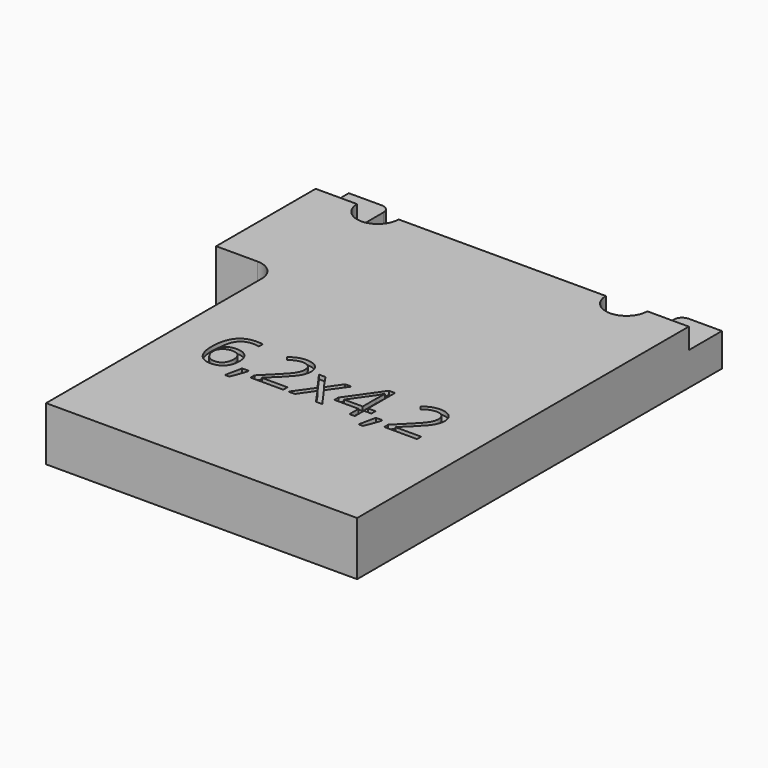
from build123d import *

# Parameters (mm, degrees)
F1_DEPTH     = 13
F2_W         = 107.3082715438
F2_H         = 14.5000026375
F3_DEPTH     = 5
F4_R         = 3
F5_DEPTH     = 10
F6_TEXT_SIZE = 16.861082986
F7_DEPTH     = 1


# Not quite as in the source:
# - Text() gives the source's letters only with a copy of the font that has no kerning and outlines rounded to 1/6400 em; it was checked with that copy


with BuildPart() as f1:
    # F0 (on Top) → F1 (new body)
    with BuildSketch(Plane.XY):
        with BuildLine():
            Line((-42.4800007343, 29.9199996144), (-42.4800007343, -10.0800003856))
            Line((-42.4800007343, -10.0800003856), (-32.5100003928, -10.0800003856))
            ThreePointArc((-32.5100003928, -10.0800003856), (-28.9744664869, -11.5444664797), (-27.5100003928, -15.0800003856))
            Line((-27.5100003928, -15.0800003856), (-27.5100003928, -80.0800003856))
            Line((-27.5100003928, -80.0800003856), (47.5199992657, -80.0800003856))
            Line((47.5199992657, -80.0800003856), (47.5199992657, 29.9199996144))
            Line((47.5199992657, 29.9199996144), (39.5199992657, 29.9199996144))
            ThreePointArc((39.5199992657, 29.9199996144), (38.1057857033, 29.3342131767), (37.5199992657, 27.9199996144))
            Line((37.5199992657, 27.9199996144), (37.5199992657, 19.9199996144))
            ThreePointArc((37.5199992657, 19.9199996144), (32.5199992657, 14.9199996144), (27.5199992657, 19.9199996144))
            Line((27.5199992657, 19.9199996144), (-22.4800007343, 19.9199996144))
            ThreePointArc((-22.4800007343, 19.9199996144), (-27.4800007343, 14.9199996144), (-32.4800007343, 19.9199996144))
            Line((-32.4800007343, 19.9199996144), (-32.4800007343, 27.9199996144))
            ThreePointArc((-32.4800007343, 27.9199996144), (-33.065787172, 29.3342131767), (-34.4800007343, 29.9199996144))
            Line((-34.4800007343, 29.9199996144), (-42.4800007343, 29.9199996144))
        make_face()
    extrude(amount=F1_DEPTH)

    # F2 (on face) → F3 (cut)
    with BuildSketch(Plane.XY.offset(13)):
        with Locations((10.5722389322, 27.1700009331)):
            Rectangle(F2_W, F2_H)
    extrude(amount=-F3_DEPTH, mode=Mode.SUBTRACT)

    # F4 (on face) → F5 (cut)
    with BuildSketch(Plane(origin=(0, 19.9199996144, 0), x_dir=(-1, 0, 0), z_dir=(0, 1, 0))):
        with Locations((-17.5199992657, 6.5)):
            Circle(F4_R)
    extrude(amount=-F5_DEPTH, mode=Mode.SUBTRACT)

    # F6 (on face) → F7 (cut)
    with BuildSketch(Plane.XY.offset(13)):
        with Locations((-18.5406059027, -47.8933230042)):
            Text('6,2x4,2', F6_TEXT_SIZE, font='Open Sans', text_align=(TextAlign.LEFT, TextAlign.BOTTOM))
    extrude(amount=-F7_DEPTH, mode=Mode.SUBTRACT)


solid = f1.part
